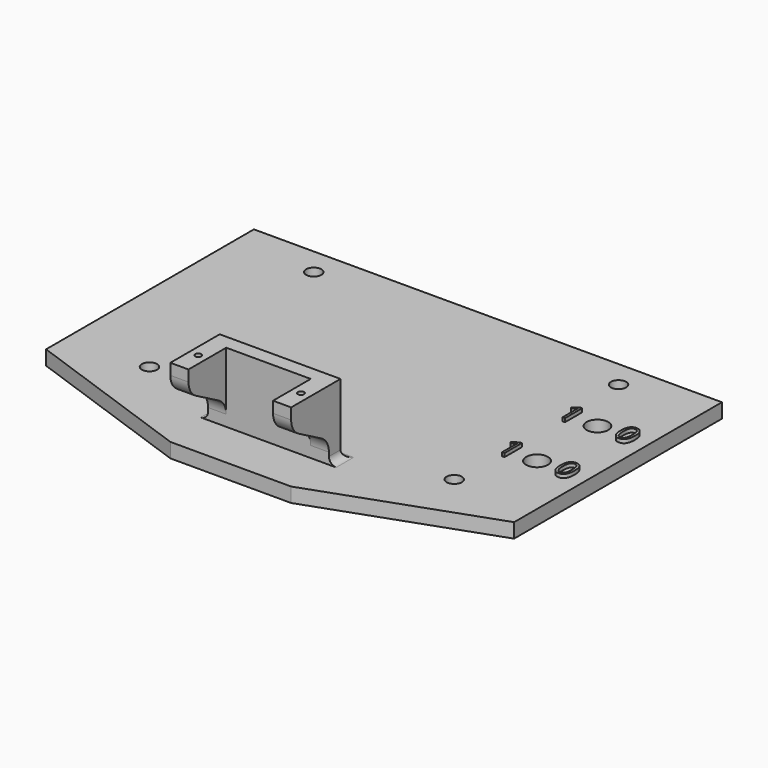
from build123d import *

# Parameters (mm, degrees)
F1_W         = 5
F1_H         = 7.2
F1_H_2       = 6
F1_H_3       = 4
F1_W_2       = 23.3
F3_DEPTH     = 8.5
F0_W         = 23.3
F0_H         = 4
F4_DEPTH     = 23.2
F5_DEPTH     = 18.1
F6_START     = 4.3
F0_R         = 0.85
F6_DEPTH     = 20.7
F7_R         = 2.1
F7_W         = 129
F7_H         = 35.8
F7_TEXT_SIZE = 8.3333333333
F8_DEPTH     = 4
F9_DEPTH     = 5
F10_R        = 2


# Not quite as in the source:
# - Text() gives the source's letters only with a copy of the font that has no kerning and outlines rounded to 1/6400 em; it was checked with that copy


with BuildPart() as f3:
    # F1 (on Front) → F3 (new body, symmetric)
    with BuildSketch(Plane.XZ):
        with Locations((-14.15, 13.6)):
            Rectangle(F1_W, F1_H)
        with Locations((-14.15, 20.2)):
            Rectangle(F1_W, F1_H_2)
        with Locations((-14.15, 7)):
            Rectangle(F1_W, F1_H_2)
        with Locations((-14.15, 2)):
            Rectangle(F1_W, F1_H_3)
        with Locations((0, 2)):
            Rectangle(F1_W_2, F1_H_3)
        with Locations((14.15, 2)):
            Rectangle(F1_W, F1_H_3)
        with Locations((14.15, 7)):
            Rectangle(F1_W, F1_H_2)
        with Locations((14.15, 13.6)):
            Rectangle(F1_W, F1_H)
        with Locations((14.15, 20.2)):
            Rectangle(F1_W, F1_H_2)
    extrude(amount=F3_DEPTH, both=True)

    # F0 (on Top) → F4 (join)
    with BuildSketch(Plane.XY):
        with Locations((0, 6.5)):
            Rectangle(F0_W, F0_H)
    extrude(amount=F4_DEPTH)

    # F2 (on Right) → F5 (cut, symmetric)
    with BuildSketch(Plane.YZ):
        with BuildLine():
            Line((-8.5, 17.2), (-8.5, 10))
            Line((-8.5, 10), (3.5396314061, 10))
            ThreePointArc((3.5396314061, 10), (2.8089650426, 10.8020152096), (1.9224991399, 11.4275389379))
            Line((1.9224991399, 11.4275389379), (-5.9224991399, 15.7724610621))
            ThreePointArc((-5.9224991399, 15.7724610621), (-6.8089650426, 16.3979847904), (-7.5396314061, 17.2))
            Line((-7.5396314061, 17.2), (-8.5, 17.2))
        make_face()
        with BuildLine():
            Line((-8.5, 20.1464178425), (-8.5, 17.2))
            Line((-8.5, 17.2), (-7.5396314061, 17.2))
            ThreePointArc((-7.5396314061, 17.2), (-8.2538488107, 18.5969271247), (-8.5, 20.1464178425))
        make_face()
        with BuildLine():
            Line((-8.5, 10), (-8.5, 4))
            Line((-8.5, 4), (4.5, 4))
            Line((4.5, 4), (4.5, 7.0535821575))
            ThreePointArc((4.5, 7.0535821575), (4.2538488107, 8.6030728753), (3.5396314061, 10))
            Line((3.5396314061, 10), (-8.5, 10))
        make_face()
    extrude(amount=F5_DEPTH, both=True, mode=Mode.SUBTRACT)

    # F0 (on Top) → F6 (cut)
    with BuildSketch(Plane.XY.offset(F6_START)):
        with Locations((14.15, -2)):
            Circle(F0_R)
        with Locations((-14.15, -2)):
            Circle(F0_R)
    extrude(amount=F6_DEPTH, mode=Mode.SUBTRACT)

    # F7 (on Top) → F8 (join)
    with BuildSketch(Plane.XY):
        Polygon((64.5, 44.3), (-64.5, 44.3), (-64.5, 8.5), (0, 8.5), (64.5, 8.5), align=None)
        with Locations((-42, 16)):
            Circle(F7_R, mode=Mode.SUBTRACT)
        with Locations((42, 16)):
            Circle(F7_R, mode=Mode.SUBTRACT)
        with BuildLine():
            Line((43.9596354167, 36.84921875), (43.9596354167, 30.9))
            Line((43.9596354167, 30.9), (43.30078125, 30.9))
            Line((43.30078125, 30.9), (43.30078125, 35.1395833333))
            add(Edge.make_bspline(
                [(43.30078125, 35.1395833333), (43.30078125, 35.66953125), (43.3333333333, 36.1408854167)],
                knots=[0, 0, 0, 1, 1, 1], degree=2))
            add(Edge.make_bspline(
                [(43.3333333333, 36.1408854167), (43.2486979167, 36.0549479167), (43.142578125, 35.9618489583)],
                knots=[0, 0, 0, 1, 1, 1], degree=2))
            add(Edge.make_bspline(
                [(43.142578125, 35.9618489583), (43.0364583333, 35.86875), (42.1744791667, 35.1682291667)],
                knots=[0, 0, 0, 1, 1, 1], degree=2))
            Line((42.1744791667, 35.1682291667), (41.81640625, 35.6317708333))
            Line((41.81640625, 35.6317708333), (43.390625, 36.84921875))
            Line((43.390625, 36.84921875), (43.9596354167, 36.84921875))
        make_face(mode=Mode.SUBTRACT)
        with BuildLine():
            ThreePointArc((47.5, 33.9), (50.5, 36.9), (53.5, 33.9))
            ThreePointArc((53.5, 33.9), (50.5, 30.9), (47.5, 33.9))
        make_face(mode=Mode.SUBTRACT)
        with BuildLine():
            add(Edge.make_bspline(
                [(60.34765625, 36.1571614583), (60.8502604167, 35.3713541667), (60.8502604167, 33.8830729167)],
                knots=[0, 0, 0, 1, 1, 1], degree=2))
            add(Edge.make_bspline(
                [(60.8502604167, 33.8830729167), (60.8502604167, 32.3401041667), (60.3639322917, 31.5790364583)],
                knots=[0, 0, 0, 1, 1, 1], degree=2))
            add(Edge.make_bspline(
                [(60.3639322917, 31.5790364583), (59.8776041667, 30.81796875), (58.8763020833, 30.81796875)],
                knots=[0, 0, 0, 1, 1, 1], degree=2))
            add(Edge.make_bspline(
                [(58.8763020833, 30.81796875), (57.9166666667, 30.81796875), (57.416015625, 31.597265625)],
                knots=[0, 0, 0, 1, 1, 1], degree=2))
            add(Edge.make_bspline(
                [(57.416015625, 31.597265625), (56.9153645833, 32.3765625), (56.9153645833, 33.8830729167)],
                knots=[0, 0, 0, 1, 1, 1], degree=2))
            add(Edge.make_bspline(
                [(56.9153645833, 33.8830729167), (56.9153645833, 35.4364583333), (57.3997395833, 36.1897135417)],
                knots=[0, 0, 0, 1, 1, 1], degree=2))
            add(Edge.make_bspline(
                [(57.3997395833, 36.1897135417), (57.8841145833, 36.94296875), (58.8763020833, 36.94296875)],
                knots=[0, 0, 0, 1, 1, 1], degree=2))
            add(Edge.make_bspline(
                [(58.8763020833, 36.94296875), (59.8450520833, 36.94296875), (60.34765625, 36.1571614583)],
                knots=[0, 0, 0, 1, 1, 1], degree=2))
        make_face(mode=Mode.SUBTRACT)
        with Locations((0, 62.2)):
            Rectangle(F7_W, F7_H)
        with Locations((-42, 72.6)):
            Circle(F7_R, mode=Mode.SUBTRACT)
        with BuildLine():
            Line((43.9596354167, 57.64921875), (43.9596354167, 51.7))
            Line((43.9596354167, 51.7), (43.30078125, 51.7))
            Line((43.30078125, 51.7), (43.30078125, 55.9395833333))
            add(Edge.make_bspline(
                [(43.30078125, 55.9395833333), (43.30078125, 56.46953125), (43.3333333333, 56.9408854167)],
                knots=[0, 0, 0, 1, 1, 1], degree=2))
            add(Edge.make_bspline(
                [(43.3333333333, 56.9408854167), (43.2486979167, 56.8549479167), (43.142578125, 56.7618489583)],
                knots=[0, 0, 0, 1, 1, 1], degree=2))
            add(Edge.make_bspline(
                [(43.142578125, 56.7618489583), (43.0364583333, 56.66875), (42.1744791667, 55.9682291667)],
                knots=[0, 0, 0, 1, 1, 1], degree=2))
            Line((42.1744791667, 55.9682291667), (41.81640625, 56.4317708333))
            Line((41.81640625, 56.4317708333), (43.390625, 57.64921875))
            Line((43.390625, 57.64921875), (43.9596354167, 57.64921875))
        make_face(mode=Mode.SUBTRACT)
        with BuildLine():
            ThreePointArc((47.5, 54.7), (50.5, 57.7), (53.5, 54.7))
            ThreePointArc((53.5, 54.7), (50.5, 51.7), (47.5, 54.7))
        make_face(mode=Mode.SUBTRACT)
        with BuildLine():
            add(Edge.make_bspline(
                [(60.34765625, 56.9571614583), (60.8502604167, 56.1713541667), (60.8502604167, 54.6830729167)],
                knots=[0, 0, 0, 1, 1, 1], degree=2))
            add(Edge.make_bspline(
                [(60.8502604167, 54.6830729167), (60.8502604167, 53.1401041667), (60.3639322917, 52.3790364583)],
                knots=[0, 0, 0, 1, 1, 1], degree=2))
            add(Edge.make_bspline(
                [(60.3639322917, 52.3790364583), (59.8776041667, 51.61796875), (58.8763020833, 51.61796875)],
                knots=[0, 0, 0, 1, 1, 1], degree=2))
            add(Edge.make_bspline(
                [(58.8763020833, 51.61796875), (57.9166666667, 51.61796875), (57.416015625, 52.397265625)],
                knots=[0, 0, 0, 1, 1, 1], degree=2))
            add(Edge.make_bspline(
                [(57.416015625, 52.397265625), (56.9153645833, 53.1765625), (56.9153645833, 54.6830729167)],
                knots=[0, 0, 0, 1, 1, 1], degree=2))
            add(Edge.make_bspline(
                [(56.9153645833, 54.6830729167), (56.9153645833, 56.2364583333), (57.3997395833, 56.9897135417)],
                knots=[0, 0, 0, 1, 1, 1], degree=2))
            add(Edge.make_bspline(
                [(57.3997395833, 56.9897135417), (57.8841145833, 57.74296875), (58.8763020833, 57.74296875)],
                knots=[0, 0, 0, 1, 1, 1], degree=2))
            add(Edge.make_bspline(
                [(58.8763020833, 57.74296875), (59.8450520833, 57.74296875), (60.34765625, 56.9571614583)],
                knots=[0, 0, 0, 1, 1, 1], degree=2))
        make_face(mode=Mode.SUBTRACT)
        with Locations((42, 72.6)):
            Circle(F7_R, mode=Mode.SUBTRACT)
        Polygon((0, 8.5), (-64.5, 8.5), (-16.65, -8.5), (16.65, -8.5), (64.5, 8.5), align=None)
        with Locations((56.5, 30.9)):
            Text('0', F7_TEXT_SIZE, font='Open Sans', text_align=(TextAlign.LEFT, TextAlign.BOTTOM))
        with Locations((56.5, 51.7)):
            Text('0', F7_TEXT_SIZE, font='Open Sans', text_align=(TextAlign.LEFT, TextAlign.BOTTOM))
        with BuildLine():
            add(Edge.make_bspline(
                [(57.904296875, 35.769140625), (57.5989583333, 35.18125), (57.5989583333, 33.8830729167)],
                knots=[0, 0, 0, 1, 1, 1], degree=2))
            add(Edge.make_bspline(
                [(57.5989583333, 33.8830729167), (57.5989583333, 32.5848958333), (57.904296875, 31.9924479167)],
                knots=[0, 0, 0, 1, 1, 1], degree=2))
            add(Edge.make_bspline(
                [(57.904296875, 31.9924479167), (58.2096354167, 31.4), (58.8763020833, 31.4)],
                knots=[0, 0, 0, 1, 1, 1], degree=2))
            add(Edge.make_bspline(
                [(58.8763020833, 31.4), (59.5520833333, 31.4), (59.8548177083, 32.0002604167)],
                knots=[0, 0, 0, 1, 1, 1], degree=2))
            add(Edge.make_bspline(
                [(59.8548177083, 32.0002604167), (60.1575520833, 32.6005208333), (60.1575520833, 33.8830729167)],
                knots=[0, 0, 0, 1, 1, 1], degree=2))
            add(Edge.make_bspline(
                [(60.1575520833, 33.8830729167), (60.1575520833, 35.1643229167), (59.8548177083, 35.7606770833)],
                knots=[0, 0, 0, 1, 1, 1], degree=2))
            add(Edge.make_bspline(
                [(59.8548177083, 35.7606770833), (59.5520833333, 36.35703125), (58.8763020833, 36.35703125)],
                knots=[0, 0, 0, 1, 1, 1], degree=2))
            add(Edge.make_bspline(
                [(58.8763020833, 36.35703125), (58.2096354167, 36.35703125), (57.904296875, 35.769140625)],
                knots=[0, 0, 0, 1, 1, 1], degree=2))
        make_face()
        with BuildLine():
            add(Edge.make_bspline(
                [(57.904296875, 56.569140625), (57.5989583333, 55.98125), (57.5989583333, 54.6830729167)],
                knots=[0, 0, 0, 1, 1, 1], degree=2))
            add(Edge.make_bspline(
                [(57.5989583333, 54.6830729167), (57.5989583333, 53.3848958333), (57.904296875, 52.7924479167)],
                knots=[0, 0, 0, 1, 1, 1], degree=2))
            add(Edge.make_bspline(
                [(57.904296875, 52.7924479167), (58.2096354167, 52.2), (58.8763020833, 52.2)],
                knots=[0, 0, 0, 1, 1, 1], degree=2))
            add(Edge.make_bspline(
                [(58.8763020833, 52.2), (59.5520833333, 52.2), (59.8548177083, 52.8002604167)],
                knots=[0, 0, 0, 1, 1, 1], degree=2))
            add(Edge.make_bspline(
                [(59.8548177083, 52.8002604167), (60.1575520833, 53.4005208333), (60.1575520833, 54.6830729167)],
                knots=[0, 0, 0, 1, 1, 1], degree=2))
            add(Edge.make_bspline(
                [(60.1575520833, 54.6830729167), (60.1575520833, 55.9643229167), (59.8548177083, 56.5606770833)],
                knots=[0, 0, 0, 1, 1, 1], degree=2))
            add(Edge.make_bspline(
                [(59.8548177083, 56.5606770833), (59.5520833333, 57.15703125), (58.8763020833, 57.15703125)],
                knots=[0, 0, 0, 1, 1, 1], degree=2))
            add(Edge.make_bspline(
                [(58.8763020833, 57.15703125), (58.2096354167, 57.15703125), (57.904296875, 56.569140625)],
                knots=[0, 0, 0, 1, 1, 1], degree=2))
        make_face()
        with Locations((41.05078125, 30.9)):
            Text('1', F7_TEXT_SIZE, font='Open Sans', text_align=(TextAlign.LEFT, TextAlign.BOTTOM))
        with Locations((41.05078125, 51.7)):
            Text('1', F7_TEXT_SIZE, font='Open Sans', text_align=(TextAlign.LEFT, TextAlign.BOTTOM))
    extrude(amount=F8_DEPTH)

    # F7 (on Top) → F9 (join)
    with BuildSketch(Plane.XY):
        with Locations((41.05078125, 30.9)):
            Text('1', F7_TEXT_SIZE, font='Open Sans', text_align=(TextAlign.LEFT, TextAlign.BOTTOM))
        with Locations((56.5, 30.9)):
            Text('0', F7_TEXT_SIZE, font='Open Sans', text_align=(TextAlign.LEFT, TextAlign.BOTTOM))
        with Locations((41.05078125, 51.7)):
            Text('1', F7_TEXT_SIZE, font='Open Sans', text_align=(TextAlign.LEFT, TextAlign.BOTTOM))
        with Locations((56.5, 51.7)):
            Text('0', F7_TEXT_SIZE, font='Open Sans', text_align=(TextAlign.LEFT, TextAlign.BOTTOM))
    extrude(amount=F9_DEPTH)

    # F10
    f10_edges = [f3.edges().sort_by_distance(p)[0] for p in [
        (0, 8.5, 4),
        (16.65, 6.5, 4),
        (-16.65, 6.5, 4),
    ]]
    fillet(f10_edges, radius=F10_R)


solid = f3.part
